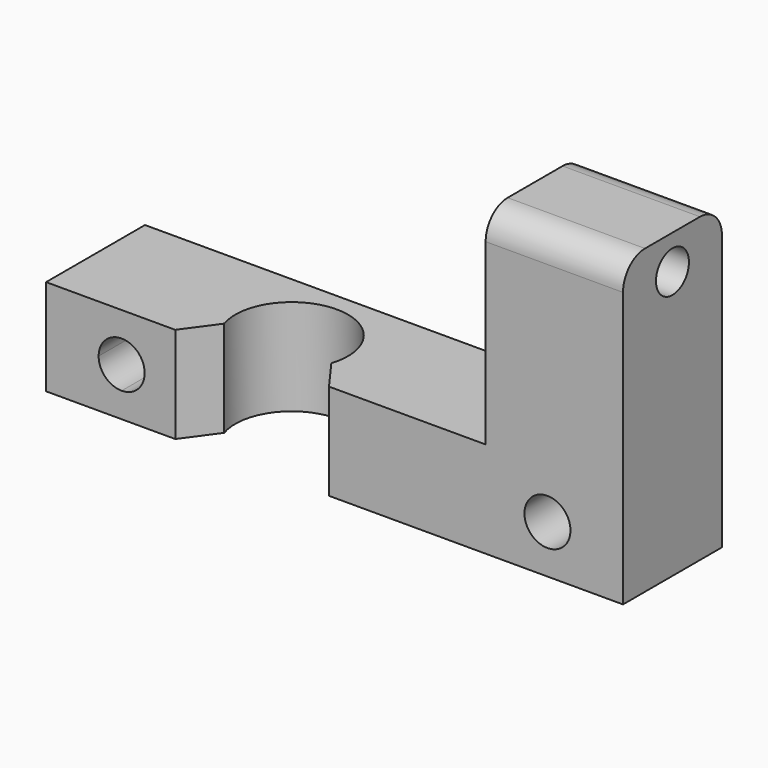
from build123d import *

# Parameters (mm, degrees)
F1_W        = 42
F1_H        = 9
F2_DEPTH    = 7
F3_R        = 4.1
F4_DEPTH    = 25
F5_T1_DEPTH = 26.0282480506
F7_DEPTH    = 25
F8_W        = 10
F8_H        = 9
F9_DEPTH    = 15
F10_R       = 1.5
F11_DEPTH   = 25
F12_R       = 2


# Not quite as in the source:
# - a fillet or chamfer that OpenCascade refuses, or shapes differently, is made with other operations: its cross-section is extruded or revolved along the edge and cut away or added


with BuildPart() as f2:
    # F1 (on Top) → F2 (new body)
    with BuildSketch(Plane.XY):
        with Locations((21, 4.5)):
            Rectangle(F1_W, F1_H)
    extrude(amount=F2_DEPTH)

    # F3 (on face) → F4 (cut)
    with BuildSketch(Plane.XY.offset(7)):
        with Locations((15, 3.6)):
            Circle(F3_R)
    extrude(amount=-F4_DEPTH, mode=Mode.SUBTRACT)

    # F5: chamfer of 7 on 2 edges, made by hand

    # F5_s2 → F5_t1 (cut)
    with BuildSketch(Plane.XY.offset(-9.5141240253)):
        with BuildLine():
            Line((20.7610452751, -0.2264961011), (18.73515334, 2.5608842714))
            Line((18.73515334, 2.5608842714), (18.6019903715, 2.6041002851))
            ThreePointArc((18.6019903715, 2.6041002851), (18.0707550937, 1.0995874031), (16.895141727, 0.1229268293))
            Line((16.895141727, 0.1229268293), (16.962141687, -0.14))
            ThreePointArc((16.962141687, -0.14), (18.861593481, -0.14), (20.7610452751, -0.3664961011))
            Line((20.7610452751, -0.3664961011), (20.7610452751, -0.2264961011))
        make_face()
        with BuildLine():
            Line((11.26484666, 2.5608842714), (9.2389547249, -0.2264961011))
            Line((9.2389547249, -0.2264961011), (9.2389547249, -0.3664961011))
            ThreePointArc((9.2389547249, -0.3664961011), (11.138406519, -0.14), (13.037858313, -0.14))
            Line((13.037858313, -0.14), (13.104858273, 0.1229268293))
            ThreePointArc((13.104858273, 0.1229268293), (11.9292449063, 1.0995874031), (11.3980096285, 2.6041002851))
            Line((11.3980096285, 2.6041002851), (11.26484666, 2.5608842714))
        make_face()
    extrude(amount=F5_T1_DEPTH, mode=Mode.SUBTRACT)

    # F6 (on face) → F7 (cut)
    with BuildSketch(Plane(origin=(0, 9, 0), x_dir=(-1, 0, 0), z_dir=(0, 1, 0))):
        with BuildLine():
            Line((-5.5, 3.5), (-3.825, 3.5))
            ThreePointArc((-3.825, 3.5), (-4.3155961415, 4.6844038585), (-5.5, 5.175))
            Line((-5.5, 5.175), (-5.5, 3.5))
        make_face()
        with BuildLine():
            ThreePointArc((-5.5, 1.825), (-4.3155961415, 2.3155961415), (-3.825, 3.5))
            Line((-3.825, 3.5), (-5.5, 3.5))
            Line((-5.5, 3.5), (-5.5, 1.825))
        make_face()
        with BuildLine():
            Line((-5.5, 3.5), (-5.5, 5.175))
            ThreePointArc((-5.5, 5.175), (-7.175, 3.5), (-5.5, 1.825))
            Line((-5.5, 1.825), (-5.5, 3.5))
        make_face()
        with BuildLine():
            ThreePointArc((-38.175, 3.5), (-36.5, 1.825), (-34.825, 3.5))
            ThreePointArc((-34.825, 3.5), (-36.5, 5.175), (-38.175, 3.5))
        make_face()
    extrude(amount=-F7_DEPTH, mode=Mode.SUBTRACT)

    # F8 (on face) → F9 (join)
    with BuildSketch(Plane.XY.offset(7)):
        with Locations((37, 4.5)):
            Rectangle(F8_W, F8_H)
    extrude(amount=F9_DEPTH)

    # F10 (on face) → F11 (cut)
    with BuildSketch(Plane.YZ.offset(42)):
        with Locations((4.5, 19.5)):
            Circle(F10_R)
    extrude(amount=-F11_DEPTH, mode=Mode.SUBTRACT)

    # F12
    f12_edges = [f2.edges().sort_by_distance(p)[0] for p in [
        (37, 0, 22),
        (37, 9, 22),
    ]]
    fillet(f12_edges, radius=F12_R)


solid = f2.part
